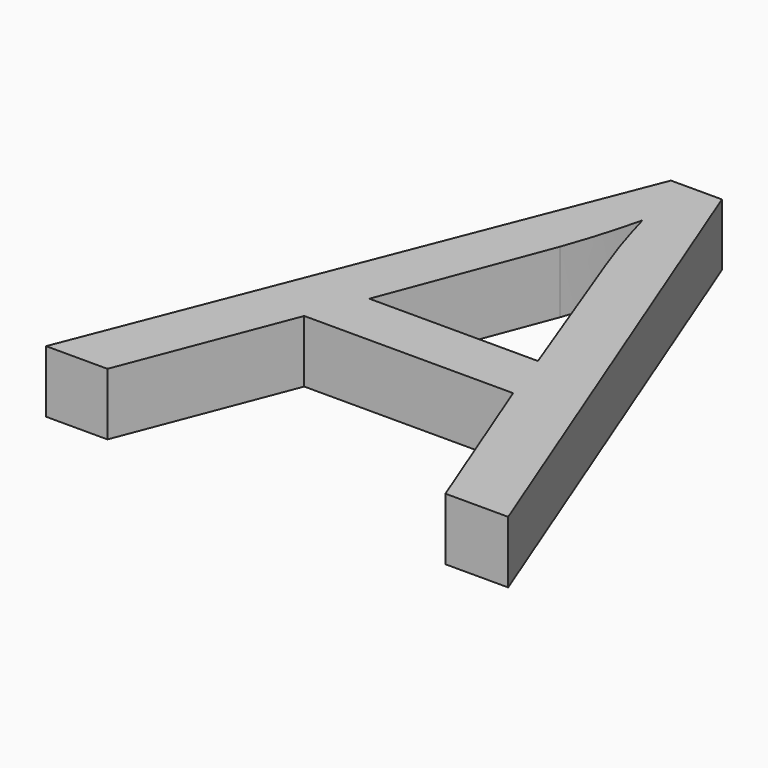
from build123d import *

# Parameters (mm, degrees)
F0_TEXT_SIZE = 74.5934537715
F1_DEPTH     = 6.35


# Not quite as in the source:
# - Text() gives the source's letters only with a copy of the font that has no kerning and outlines rounded to 1/6400 em; it was checked with that copy


with BuildPart() as f1:
    # F0 (on Top) → F1 (new body)
    with BuildSketch(Plane.XY):
        with Locations((0, 0)):
            Text('A', F0_TEXT_SIZE, font='Open Sans', text_align=(TextAlign.LEFT, TextAlign.BOTTOM))
    extrude(amount=F1_DEPTH)


solid = f1.part
